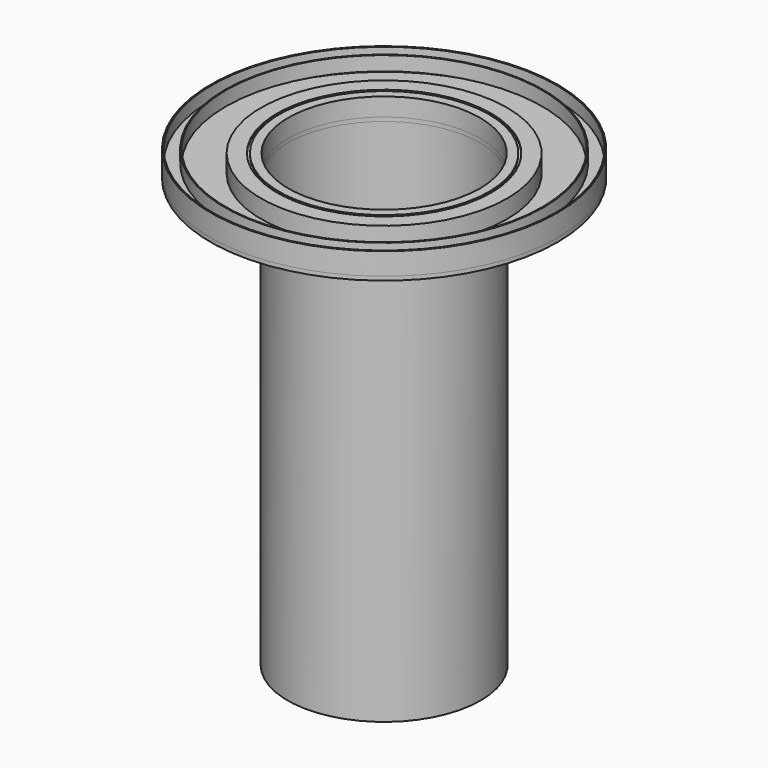
from build123d import *

# Parameters (mm, degrees)
F1_R      = 405
F1_R_2    = 370
F2_DEPTH  = 70
F3_R      = 414
F3_R_2    = 405
F4_DEPTH  = 64
F5_R      = 475
F5_R_2    = 414
F6_DEPTH  = 70
F7_R      = 670
F7_R_2    = 665
F8_DEPTH  = 85
F10_R     = 615
F10_R_2   = 611
F11_DEPTH = 55
F12_R     = 665
F12_R_2   = 615
F13_DEPTH = 5
F0_R      = 372.5
F0_R_2    = 370
F14_DEPTH = 1670
F16_R     = 670
F16_R_2   = 370
F17_DEPTH = 15


with BuildPart() as f2:
    # F1 (on face) → F2 (new body)
    with BuildSketch(Plane.XY):
        Circle(F1_R)
        Circle(F1_R_2, mode=Mode.SUBTRACT)
    extrude(amount=F2_DEPTH)


with BuildPart() as f4:
    # F3 (on face) → F4 (new body)
    with BuildSketch(Plane.XY):
        Circle(F3_R)
        Circle(F3_R_2, mode=Mode.SUBTRACT)
    extrude(amount=F4_DEPTH)


with BuildPart() as f6:
    # F5 (on face) → F6 (new body)
    with BuildSketch(Plane.XY):
        Circle(F5_R)
        Circle(F5_R_2, mode=Mode.SUBTRACT)
    extrude(amount=F6_DEPTH)


with BuildPart() as f8:
    # F7 (on face) → F8 (new body)
    with BuildSketch(Plane.XY):
        Circle(F7_R)
        Circle(F7_R_2, mode=Mode.SUBTRACT)
    extrude(amount=F8_DEPTH)


with BuildPart() as f11:
    # F10 (on offset) → F11 (new body)
    with BuildSketch(Plane.XY.offset(30)):
        Circle(F10_R)
        Circle(F10_R_2, mode=Mode.SUBTRACT)
    extrude(amount=F11_DEPTH)


with BuildPart() as f13:
    # F12 (on offset) → F13 (new body)
    with BuildSketch(Plane.XY.offset(30)):
        Circle(F12_R)
        Circle(F12_R_2, mode=Mode.SUBTRACT)
    extrude(amount=F13_DEPTH)


with BuildPart() as f14:
    # F0 (on Top) → F14 (new body)
    with BuildSketch(Plane.XY):
        Circle(F0_R)
        Circle(F0_R_2, mode=Mode.SUBTRACT)
    extrude(amount=-F14_DEPTH)


with BuildPart() as f17:
    # F16 (on offset) → F17 (new body)
    with BuildSketch(Plane.XY.offset(-15)):
        Circle(F16_R)
        Circle(F16_R_2, mode=Mode.SUBTRACT)
    extrude(amount=F17_DEPTH)


solid = Compound([f2.part, f4.part, f6.part, f8.part, f11.part, f13.part, f14.part, f17.part])
